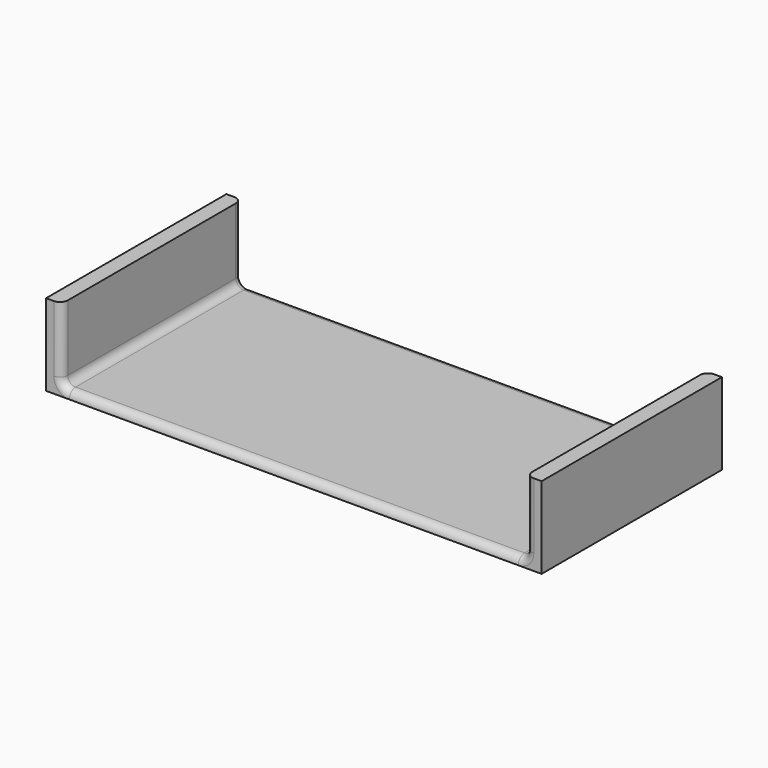
from build123d import *

# Parameters (mm, degrees)
F1_DEPTH = 58
F2_F1_R  = 2
F2_F2_R  = 1.9999


# Not quite as in the source:
# - a fillet or chamfer is up to 0.001 mm smaller than in the source, because OpenCascade refuses the exact size


with BuildPart() as f1:
    # F0 (on Front) → F1 (new body)
    with BuildSketch(Plane.XZ):
        Polygon((70.3524513997, 3.8339729243), (-49.1475486003, 3.8339729243), (-49.1475486003, 22.8339729243), (-53.1475486003, 22.8339729243), (-53.1475486003, 1.8339729243), (74.3524513997, 1.8339729243), (74.3524513997, 22.8339729243), (70.3524513997, 22.8339729243), align=None)
    extrude(amount=F1_DEPTH)

    # F2: fillet of radius 2 on 4 edges, made by hand

    # F2_f1
    f2_f1_edges = [f1.edges().sort_by_distance(p)[0] for p in [
        (70.3524513997, -29, 3.8339729243),
        (-49.1475486003, -29, 3.8339729243),
    ]]
    fillet(f2_f1_edges, radius=F2_F1_R)

    # F2_f2 (radius 2 in the source; OpenCascade refuses exactly that, so slightly less here)
    f2_f2_edges = [f1.edges().sort_by_distance(p)[0] for p in [
        (10.6024513997, 0, 3.8339729243),
        (10.6024513997, -58, 3.8339729243),
        (69.766664962, -58, 4.4197593619),
        (-48.5617621627, -58, 4.4197593619),
        (69.766664962, 0, 4.4197593619),
        (-48.5617621627, 0, 4.4197593619),
    ]]
    fillet(f2_f2_edges, radius=F2_F2_R)


solid = f1.part
